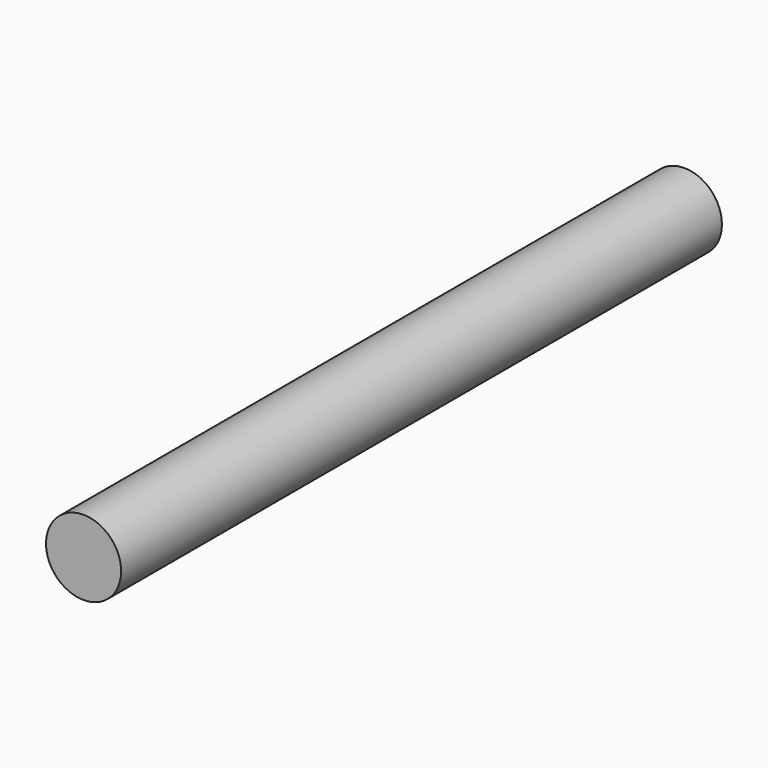
from build123d import *

# Parameters (mm, degrees)
F1_R     = 5
F2_DEPTH = 100


with BuildPart() as f2:
    # F1 (on Front) → F2 (new body)
    with BuildSketch(Plane.XZ):
        Circle(F1_R)
    extrude(amount=F2_DEPTH)


solid = f2.part
